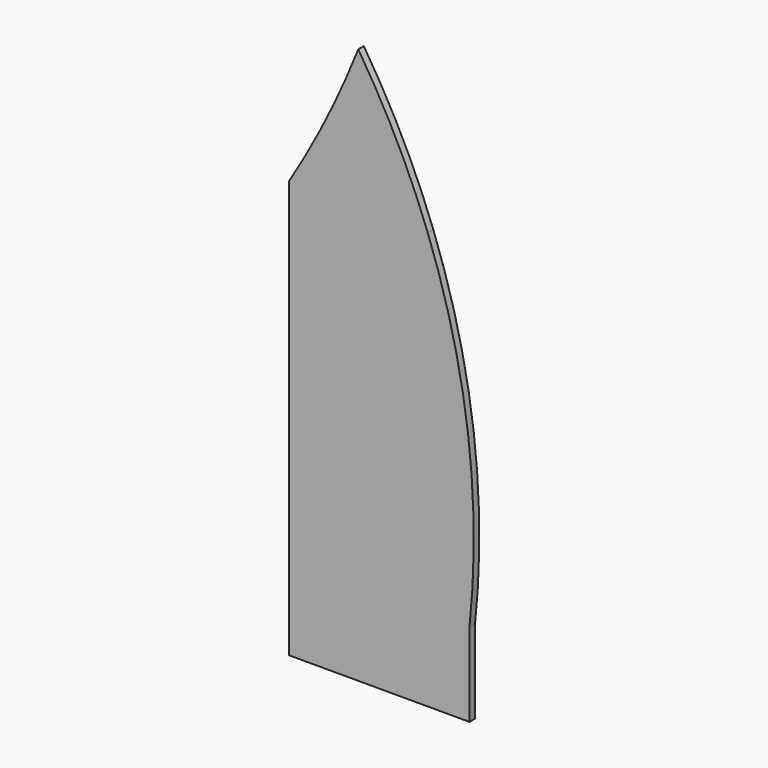
from build123d import *

# Parameters (mm, degrees)
F0_W     = 25.4
F0_H     = 203.2
F0_H_2   = 101.6
F0_W_2   = 63.5
F0_W_3   = 38.1
F1_DEPTH = 6.35


with BuildPart() as f1:
    # F0 (on Front) → F1 (new body)
    with BuildSketch(Plane.XZ):
        with Locations((12.7, 101.6)):
            Rectangle(F0_W, F0_H)
        with Locations((12.7, 254)):
            Rectangle(F0_W, F0_H_2)
        with BuildLine():
            ThreePointArc((25.4, 349.25), (13.0471808847, 326.826610923), (0, 304.8))
            Line((0, 304.8), (25.4, 304.8))
            Line((25.4, 304.8), (25.4, 349.25))
        make_face()
        with BuildLine():
            Line((25.4, 349.25), (25.4, 304.8))
            Line((25.4, 304.8), (63.5, 304.8))
            Line((63.5, 304.8), (63.5, 431.8))
            ThreePointArc((63.5, 431.8), (45.5956444739, 389.996241012), (25.4, 349.25))
        make_face()
        with BuildLine():
            Line((63.5, 431.8), (63.5, 304.8))
            Line((63.5, 304.8), (127, 304.8))
            ThreePointArc((127, 304.8), (98.6420785739, 369.996039287), (63.5, 431.8))
        make_face()
        with Locations((95.25, 254)):
            Rectangle(F0_W_2, F0_H_2)
        with Locations((44.45, 254)):
            Rectangle(F0_W_3, F0_H_2)
        Polygon((25.4, 203.2), (25.4, 0), (50.8, 0), (63.5, 0), (63.5, 203.2), align=None)
        with Locations((95.25, 101.6)):
            Rectangle(F0_W_2, F0_H)
        Polygon((152.4, 203.2), (127, 203.2), (127, 0), (130.463650802, 0), (152.4, 0), align=None)
        with BuildLine():
            Line((152.4, 0), (165.1, 0))
            ThreePointArc((165.1, 0), (168.0222390688, 35.93060895), (168.9972698039, 71.9666666667))
            ThreePointArc((168.9972698039, 71.9666666667), (158.4139149447, 190.2619875611), (127, 304.8))
            Line((127, 304.8), (127, 203.2))
            Line((127, 203.2), (152.4, 203.2))
            Line((152.4, 203.2), (152.4, 0))
        make_face()
        with BuildLine():
            Line((25.4, 0), (0, 0))
            Line((0, 0), (0, -76.2))
            Line((0, -76.2), (152.3172585759, -76.2))
            ThreePointArc((152.3172585759, -76.2), (159.8138971323, -38.2854114575), (165.1, 0))
            Line((165.1, 0), (152.4, 0))
            Line((152.4, 0), (130.463650802, 0))
            Line((130.463650802, 0), (127, 0))
            Line((127, 0), (63.5, 0))
            Line((63.5, 0), (50.8, 0))
            Line((50.8, 0), (25.4, 0))
        make_face()
        with BuildLine():
            ThreePointArc((165.1, 0), (159.8138971323, -38.2854114575), (152.3172585759, -76.2))
            Line((152.3172585759, -76.2), (165.1, -76.2))
            Line((165.1, -76.2), (165.1, 0))
        make_face()
    extrude(amount=F1_DEPTH)


solid = f1.part
